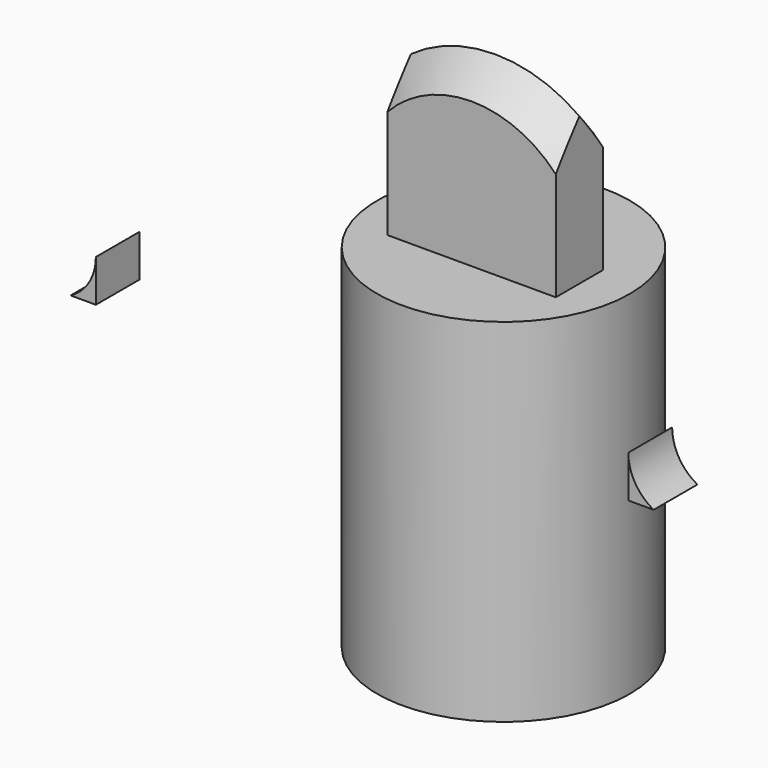
from build123d import *

# Parameters (mm, degrees)
F1_DEPTH = 7
F2_SIZE2 = 3.5
F2_SIZE  = 3.5
F3_SIZE  = 3.49999
F4_R     = 15
F5_DEPTH = 41.8
F8_DEPTH = 6.5
F9_DEPTH = 6.5


# Not quite as in the source:
# - a fillet or chamfer is up to 0.001 mm smaller than in the source, because OpenCascade refuses the exact size


with BuildPart() as f1:
    # F0 (on Front) → F1 (new body)
    with BuildSketch(Plane.XZ):
        with BuildLine():
            Line((-10, 17.5), (-10, -20.9))
            Line((-10, -20.9), (10, -20.9))
            Line((10, -20.9), (10, 17.5))
            ThreePointArc((10, 17.5), (0, 20.7252194443), (-10, 17.5))
        make_face()
    extrude(amount=F1_DEPTH)

    # F2
    f2_edges = [f1.edges().sort_by_distance(p)[0] for p in [
        (0, -7, 20.725219),
    ]]
    chamfer(f2_edges, length=F2_SIZE, length2=F2_SIZE2)

    # F3 (size 3.5 in the source; OpenCascade refuses exactly that, so slightly less here)
    f3_edges = [f1.edges().sort_by_distance(p)[0] for p in [
        (0, 0, 20.725219),
    ]]
    chamfer(f3_edges, length=F3_SIZE)


with BuildPart() as f5:
    # F4 (on Top) → F5 (new body)
    with BuildSketch(Plane.XY):
        with Locations((-0.06460234, -2.1778875962)):
            Circle(F4_R)
    extrude(amount=-F5_DEPTH)


with BuildPart() as f8:
    # F7 (on Front) → F8 (new body)
    with BuildSketch(Plane.XZ):
        with BuildLine():
            Line((18.2094871998, -13.7658946961), (18.2094871998, -18.7658946961))
            Line((18.2094871998, -18.7658946961), (21.2094871998, -18.7658946961))
            ThreePointArc((21.2094871998, -18.7658946961), (19.0170272874, -16.6813706435), (18.2094871998, -13.7658946961))
        make_face()
    extrude(amount=F8_DEPTH)


with BuildPart() as f9:
    # F6 (on Front) → F9 (new body)
    with BuildSketch(Plane.XZ):
        with BuildLine():
            ThreePointArc((-44.992926091, -13.8715998083), (-45.8004661786, -16.7870757558), (-47.992926091, -18.8715998083))
            Line((-47.992926091, -18.8715998083), (-44.992926091, -18.8715998083))
            Line((-44.992926091, -18.8715998083), (-44.992926091, -13.8715998083))
        make_face()
    extrude(amount=F9_DEPTH)


solid = Compound([f1.part, f5.part, f8.part, f9.part])
